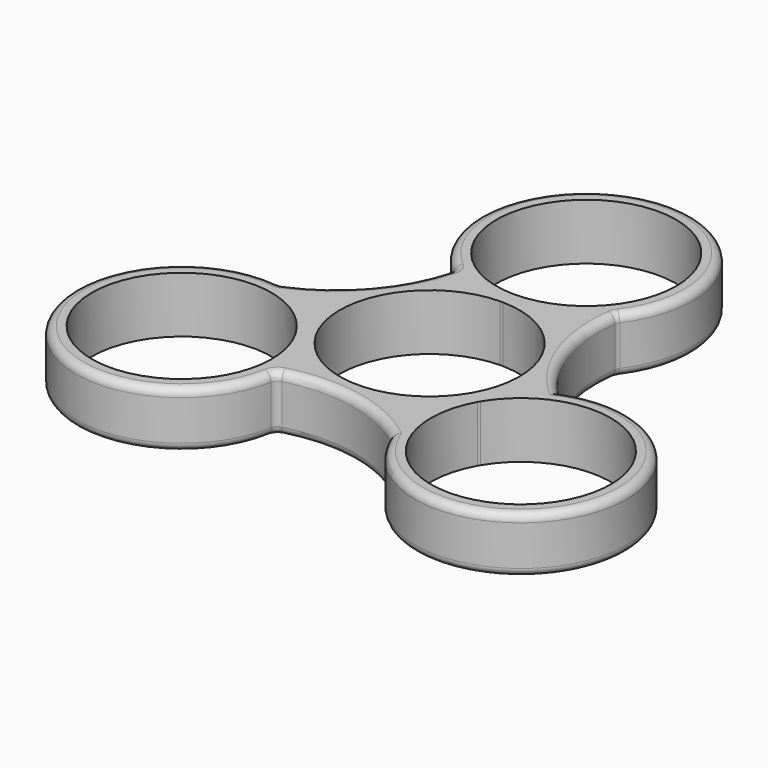
from build123d import *

# Parameters (mm, degrees)
F1_DEPTH = 7
F2_F1_R  = 1
F2_F2_R  = 1


with BuildPart() as f1:
    # F0 (on Top) → F1 (new body)
    with BuildSketch(Plane.XY):
        with BuildLine():
            ThreePointArc((16.0859033521, 0), (11.2489324437, 7.4227405942), (10.3771876201, 16.2393967891))
            ThreePointArc((10.3771876201, 16.2393967891), (-1.6415139514, 37.4949942198), (-8.042951676, 13.9308009457))
            ThreePointArc((-8.042951676, 13.9308009457), (-12.0527481421, 6.0304909646), (-19.2523239715, 0.8672097043))
            ThreePointArc((-19.2523239715, 0.8672097043), (-31.6508605334, -20.1690898925), (-8.042951676, -13.9308009457))
            ThreePointArc((-8.042951676, -13.9308009457), (0.8038156984, -13.4532315587), (8.8751363515, -17.1066064934))
            ThreePointArc((8.8751363515, -17.1066064934), (33.2923744848, -17.3259043273), (16.0859033521, 0))
        make_face()
        with BuildLine():
            ThreePointArc((-11.3427873534, -6.7513831957), (-10.2880729766, -9.3847959344), (-9.9288191789, -12.1987294406))
            ThreePointArc((-9.9288191789, -12.1987294406), (-31.9241475391, -15.1821646408), (-11.5182630349, -6.4474503999))
            ThreePointArc((-11.5182630349, -6.4474503999), (-11.4293346565, -6.5987294406), (-11.3427873534, -6.7513831957))
        make_face(mode=Mode.SUBTRACT)
        with BuildLine():
            ThreePointArc((11.5182630349, -6.4474503999), (24.1122543791, -1.4034010803), (32.3288191789, -12.1987294406))
            ThreePointArc((32.3288191789, -12.1987294406), (18.3148856726, -23.0394756429), (11.3427873534, -6.7513831957))
            ThreePointArc((11.3427873534, -6.7513831957), (11.4293346565, -6.5987294406), (11.5182630349, -6.4474503999))
        make_face(mode=Mode.SUBTRACT)
        with BuildLine():
            ThreePointArc((0.1754756815, 11.1986252855), (9.6994845224, 5.6), (9.7860318255, -5.4473462448))
            ThreePointArc((9.7860318255, -5.4473462448), (9.6972838489, -5.5987294406), (9.610556144, -5.7512790407))
            ThreePointArc((9.610556144, -5.7512790407), (0, -11.2), (-9.610556144, -5.7512790407))
            ThreePointArc((-9.610556144, -5.7512790407), (-9.6994845224, -5.6), (-9.7860318255, -5.4473462448))
            ThreePointArc((-9.7860318255, -5.4473462448), (-9.6994845224, 5.6), (-0.1754756815, 11.1986252855))
            ThreePointArc((-0.1754756815, 11.1986252855), (0, 11.2), (0.1754756815, 11.1986252855))
        make_face(mode=Mode.SUBTRACT)
        with BuildLine():
            ThreePointArc((11.2, 24.3974588811), (7.9813948541, 16.540147879), (0.1754756815, 13.1988335956))
            ThreePointArc((0.1754756815, 13.1988335956), (0, 13.1974588811), (-0.1754756815, 13.1988335956))
            ThreePointArc((-0.1754756815, 13.1988335956), (-7.8573110021, 32.3788537352), (11.2, 24.3974588811))
        make_face(mode=Mode.SUBTRACT)
    extrude(amount=F1_DEPTH)

    # F2: fillet of radius 1 on 13 edges, made by hand

    # F2_f1
    f2_f1_edges = [f1.edges().sort_by_distance(p)[0] for p in [
        (-19.2523239715, 0.8672097043, 3.5),
        (-8.042951676, -13.9308009457, 3.5),
        (10.3771876201, 16.2393967891, 3.5),
        (-8.042951676, 13.9308009457, 3.5),
    ]]
    fillet(f2_f1_edges, radius=F2_F1_R)

    # F2_f2
    f2_f2_edges = [f1.edges().sort_by_distance(p)[0] for p in [
        (-1.4628843961, 37.5161466678, 7),
        (-12.1783667806, 5.8856047573, 7),
        (-31.7584938684, -20.0249683837, 7),
        (1.1268180842, -13.5168166887, 7),
        (33.2923744848, -17.3259043273, 7),
        (11.2949912973, 7.2932435583, 7),
        (-31.7584938684, -20.0249683837, 0),
        (-1.4628843961, 37.5161466678, 0),
        (33.2923744848, -17.3259043273, 0),
        (10.4063759445, 16.2179925947, 0),
        (-8.2145805341, 13.8519992281, 0),
        (-19.2483815575, 0.9031896319, 0),
        (-7.8888929577, -14.040035038, 0),
        (10.4063759445, 16.2179925947, 7),
        (-7.8888929577, -14.040035038, 7),
        (-19.2483815575, 0.9031896319, 7),
        (-8.2145805341, 13.8519992281, 7),
    ]]
    fillet(f2_f2_edges, radius=F2_F2_R)


solid = f1.part
